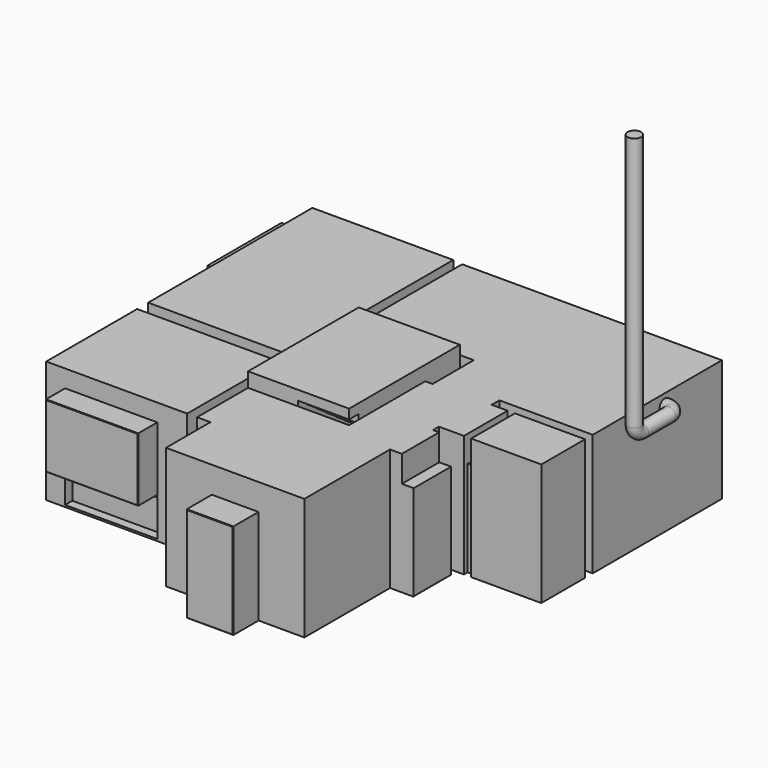
from build123d import *

# Parameters (mm, degrees)
F0_W          = 3096
F0_H          = 4507
F1_DEPTH      = 2680
F2_W          = 2025
F2_H          = 1400
F3_DEPTH      = 532
F4_W          = 2025
F4_H          = 1400
F5_DEPTH      = 532
F6_W          = 2025
F6_H          = 800
F7_DEPTH      = 200
F8_W          = 2700
F8_H          = 303
F9_DEPTH      = 2100
F11_DEPTH     = 2680
F12_W         = 219
F12_H         = 1346
F13_DEPTH     = 2100
F14_W         = 2025
F14_H         = 1400
F15_DEPTH     = 532
F17_DEPTH     = 2680
F18_W         = 1025
F18_H         = 698
F19_DEPTH     = 2100
F21_DEPTH     = 3000
F23_DEPTH     = 1110
F25_DEPTH     = 1120
F27_DEPTH     = 2680
F28_W         = 2000
F28_H         = 1400
F29_DEPTH     = 532
F30_W         = 825
F30_H         = 2100
F31_DEPTH     = 160
F32_W         = 1200
F32_H         = 2680
F33_DEPTH     = 1540
F36_W         = 1025
F36_H         = 2100
F37_DEPTH     = 260
F38_SIZE      = 10
F39_SIZE      = 10
F41_T1_DEPTH  = 2076.4336597593
F41_T3_DEPTH  = 2076.4336597593
F41_T5_DEPTH  = 2051.4336597593
F41_T7_DEPTH  = 1076.4336597593
F41_T9_DEPTH  = 1451.4336597593
F41_T11_DEPTH = 1451.4336597593
F41_T13_DEPTH = 2076.4336597593
F41_T15_DEPTH = 1441.4336597593
F41_T17_DEPTH = 2047.5714172042
F41_T19_DEPTH = 2141.4336597593
F41_T21_DEPTH = 1076.4336597593
F42_W         = 2025
F42_H         = 30
F43_DEPTH     = 200
F44_W         = 2000
F44_H         = 30
F45_DEPTH     = 200
F46_W         = 2025
F46_H         = 30
F47_DEPTH     = 180
F40_W         = 2025
F40_H         = 800
F49_DEPTH     = 200
F50_W         = 2025
F50_H         = 30
F51_DEPTH     = 200
F52_W         = 2025
F52_H         = 800
F53_DEPTH     = 200
F54_W         = 2000
F54_H         = 800
F55_DEPTH     = 200
F48_R         = 150


# Not quite as in the source:
# - a fillet or chamfer that OpenCascade refuses, or shapes differently, is made with other operations: its cross-section is extruded or revolved along the edge and cut away or added


with BuildPart() as f1:
    # F0 (on Top) → F1 (new body)
    with BuildSketch(Plane.XY):
        with Locations((-1.1402405798, 1181.2281365744)):
            Rectangle(F0_W, F0_H)
    extrude(amount=F1_DEPTH)

    # F2 (on face) → F3 (join)
    with BuildSketch(Plane(origin=(0, 3434.7281365744, 0), x_dir=(-1, 0, 0), z_dir=(0, 1, 0))):
        with Locations((-1.3597594202, 1600)):
            Rectangle(F2_W, F2_H)
    extrude(amount=F3_DEPTH)

    # F4 (on face) → F5 (join)
    with BuildSketch(Plane(origin=(-1549.1402405798, 0, 0), x_dir=(0, -1, 0), z_dir=(-1, 0, 0))):
        with Locations((-2226.2281365744, 1600)):
            Rectangle(F4_W, F4_H)
    extrude(amount=F5_DEPTH)

    # F6 (on face) → F7 (cut)
    with BuildSketch(Plane(origin=(0, 3434.7281365744, 0), x_dir=(-1, 0, 0), z_dir=(0, 1, 0))):
        with Locations((-1.3597594202, 435)):
            Rectangle(F6_W, F6_H)
    extrude(amount=-F7_DEPTH, mode=Mode.SUBTRACT)

    # F8 (on face) → F9 (join)
    with BuildSketch(Plane(origin=(0, 0, 0), x_dir=(1, 0, 0), z_dir=(0, 0, -1))):
        with Locations((-1.1402405798, 1223.7718634256)):
            Rectangle(F8_W, F8_H)
    extrude(amount=-F9_DEPTH)

    # F10 (on face) → F11 (join)
    with BuildSketch(Plane(origin=(0, 0, 0), x_dir=(1, 0, 0), z_dir=(0, 0, -1))):
        Polygon((-1549.1402405798, 3872.2718634256), (-1549.1402405798, 1375.2718634256), (-1351.1402405798, 1375.2718634256), (1546.8597594202, 1375.2718634256), (1546.8597594202, 3872.2718634256), align=None)
    extrude(amount=-F11_DEPTH)

    # F12 (on face) → F13 (join)
    with BuildSketch(Plane(origin=(0, 0, 0), x_dir=(1, 0, 0), z_dir=(0, 0, -1))):
        with Locations((1656.3597594202, 3199.2718634256)):
            Rectangle(F12_W, F12_H)
    extrude(amount=-F13_DEPTH)

    # F14 (on face) → F15 (join)
    with BuildSketch(Plane.XZ.offset(3872.2718634256)):
        with Locations((-121.6547704638, 1596.5273075876)):
            Rectangle(F14_W, F14_H)
    extrude(amount=F15_DEPTH)

    # F16 (on face) → F17 (join)
    with BuildSketch(Plane(origin=(0, 0, 0), x_dir=(1, 0, 0), z_dir=(0, 0, -1))):
        Polygon((2057.8597594202, 3872.2718634256), (1765.8597594202, 3872.2718634256), (1765.8597594202, 2526.2718634256), (1765.8597594202, 2474.2718634256), (2915.8597594202, 2474.2718634256), (2915.8597594202, 2739.2718634256), (5096.8597594202, 2739.2718634256), (5096.8597594202, 5091.2718634256), (2057.8597594202, 5091.2718634256), align=None)
    extrude(amount=-F17_DEPTH)

    # F18 (on face) → F19 (join)
    with BuildSketch(Plane(origin=(0, 0, 0), x_dir=(1, 0, 0), z_dir=(0, 0, -1))):
        with Locations((3577.3597594202, 5440.2718634256)):
            Rectangle(F18_W, F18_H)
    extrude(amount=-F19_DEPTH)

    # F20 (on face) → F21 (join)
    with BuildSketch(Plane(origin=(0, 0, 0), x_dir=(1, 0, 0), z_dir=(0, 0, -1))):
        Polygon((2915.8597594202, 2474.2718634256), (1765.8597594202, 2474.2718634256), (1765.8597594202, -565.7281365744), (3985.8597594202, -565.7281365744), (3985.8597594202, 2474.2718634256), align=None)
    extrude(amount=-F21_DEPTH)

    # F22 (on face) → F23 (cut)
    with BuildSketch(Plane(origin=(1765.8597594202, 0, 0), x_dir=(0, -1, 0), z_dir=(-1, 0, 0))):
        Polygon((1199.2718634256, 850), (1199.2718634256, 1020), (944.2718634256, 1020), (944.2718634256, 1190), (689.2718634256, 1190), (689.2718634256, 1330), (434.2718634256, 1330), (434.2718634256, 1530), (-565.7281365744, 1530), (-565.7281365744, 1330), (179.2718634256, 1330), (2219.2718634256, 0), (2474.2718634256, 0), (2474.2718634256, 170), (2219.2718634256, 170), (2219.2718634256, 340), (1964.2718634256, 340), (1964.2718634256, 510), (1709.2718634256, 510), (1709.2718634256, 680), (1454.2718634256, 680), (1454.2718634256, 850), align=None)
    extrude(amount=-F23_DEPTH, mode=Mode.SUBTRACT)

    # F24 (on face) → F25 (cut)
    with BuildSketch(Plane.YZ.offset(3985.8597594202)):
        Polygon((565.7281365744, 1330), (565.7281365744, 1530), (-689.2718634256, 1530), (-689.2718634256, 1710), (-944.2718634256, 1710), (-944.2718634256, 1890), (-1199.2718634256, 1890), (-1199.2718634256, 2070), (-1454.2718634256, 2070), (-1454.2718634256, 2250), (-1709.2718634256, 2250), (-1709.2718634256, 2430), (-1964.2718634256, 2430), (-1964.2718634256, 2610), (-2219.2718634256, 2610), (-2219.2718634256, 2790), (-2474.2718634256, 2790), (-2474.2718634256, 2651.8891687657), (-689.2718634256, 1330), align=None)
    extrude(amount=-F25_DEPTH, mode=Mode.SUBTRACT)

    # F26 (on face) → F27 (join)
    with BuildSketch(Plane.XY.offset(2680)):
        Polygon((2915.8597594202, -2739.2718634256), (5096.8597594202, -2739.2718634256), (5356.8597594202, -2739.2718634256), (5356.8597594202, -1714.2718634256), (5221.8597594202, -1714.2718634256), (5221.8597594202, -1554.2718634256), (5771.8597594202, -1554.2718634256), (5771.8597594202, -1454.2718634256), (5771.8597594202, -629.2718634256), (5771.8597594202, -354.2718634256), (5421.8597594202, -354.2718634256), (5421.8597594202, -142.2718634256), (7471.8597594202, -142.2718634256), (7471.8597594202, 3404.7281365744), (6893.8597594202, 3404.7281365744), (4681.8597594202, 3404.7281365744), (1765.8597594202, 3404.7281365744), (1765.8597594202, 747.7281365744), (4146.8597594202, 747.7281365744), (4146.8597594202, -384.2718634256), (3985.8597594202, -384.2718634256), (3985.8597594202, -2474.2718634256), (2915.8597594202, -2474.2718634256), align=None)
    extrude(amount=-F27_DEPTH)

    # F28 (on face) → F29 (join)
    with BuildSketch(Plane(origin=(0, 3404.7281365744, 0), x_dir=(-1, 0, 0), z_dir=(0, 1, 0))):
        with Locations((-5883.8597594202, 1600)):
            Rectangle(F28_W, F28_H)
    extrude(amount=F29_DEPTH)

    # F30 (on face) → F31 (join)
    with BuildSketch(Plane.YZ.offset(5771.8597594202)):
        with Locations((-1041.7718634256, 1050)):
            Rectangle(F30_W, F30_H)
    extrude(amount=F31_DEPTH)

    # F32 (on face) → F33 (join)
    with BuildSketch(Plane.YZ.offset(5931.8597594202)):
        with Locations((-954.2718634256, 1340)):
            Rectangle(F32_W, F32_H)
    extrude(amount=F33_DEPTH)

    # F34: union 

    # F36 (on face) → F37 (join)
    with BuildSketch(Plane.YZ.offset(5356.8597594202)):
        with Locations((-2226.7718634256, 1050)):
            Rectangle(F36_W, F36_H)
    extrude(amount=F37_DEPTH)

    # F38
    f38_edges = [f1.edges().sort_by_distance(p)[0] for p in [
        (1.359759, 3966.728137, 900),
    ]]
    chamfer(f38_edges, length=F38_SIZE)

    # F39
    f39_edges = [f1.edges().sort_by_distance(p)[0] for p in [
        (3577.359759, -5789.271863, 0),
    ]]
    chamfer(f39_edges, length=F39_SIZE)

    # F41: chamfer of 10 on 20 edges, made by hand

    # F41_s2 → F41_t1 (cut)
    with BuildSketch(Plane.YZ.offset(-1159.8716003435)):
        Polygon((-4394.2718634256, 896.5273075876), (-4404.2718634256, 906.5273075876), (-4404.2718634256, 896.5273075876), align=None)
        Polygon((-4394.2718634256, 2296.5273075876), (-4404.2718634256, 2286.5273075876), (-4404.2718634256, 2296.5273075876), align=None)
    extrude(amount=F41_T1_DEPTH, mode=Mode.SUBTRACT)

    # F41_s4 → F41_t3 (cut)
    with BuildSketch(Plane.XZ.offset(-3264.4449664541)):
        Polygon((-2071.1402405798, 900), (-2081.1402405798, 910), (-2081.1402405798, 900), align=None)
        Polygon((-2071.1402405798, 2300), (-2081.1402405798, 2290), (-2081.1402405798, 2300), align=None)
    extrude(amount=F41_T3_DEPTH, mode=Mode.SUBTRACT)

    # F41_s6 → F41_t5 (cut)
    with BuildSketch(Plane.YZ.offset(4858.1429295405)):
        Polygon((3926.7281365744, 900), (3936.7281365744, 910), (3936.7281365744, 900), align=None)
        Polygon((3926.7281365744, 2300), (3936.7281365744, 2290), (3936.7281365744, 2300), align=None)
    extrude(amount=F41_T5_DEPTH, mode=Mode.SUBTRACT)

    # F41_s8 → F41_t7 (cut)
    with BuildSketch(Plane.XZ.offset(1688.5550335459)):
        Polygon((5606.8597594202, 0), (5616.8597594202, 10), (5616.8597594202, 0), align=None)
    extrude(amount=F41_T7_DEPTH, mode=Mode.SUBTRACT)

    # F41_s10 → F41_t9 (cut)
    with BuildSketch(Plane.XY.offset(870.8104777079)):
        Polygon((-1134.1547704638, -4394.2718634256), (-1124.1547704638, -4404.2718634256), (-1134.1547704638, -4404.2718634256), align=None)
        Polygon((890.8452295362, -4394.2718634256), (880.8452295362, -4404.2718634256), (890.8452295362, -4404.2718634256), align=None)
    extrude(amount=F41_T9_DEPTH, mode=Mode.SUBTRACT)

    # F41_s12 → F41_t11 (cut)
    with BuildSketch(Plane.XY.offset(874.2831701203)):
        Polygon((-2071.1402405798, 1213.7281365744), (-2081.1402405798, 1223.7281365744), (-2081.1402405798, 1213.7281365744), align=None)
        Polygon((-2071.1402405798, 3238.7281365744), (-2081.1402405798, 3228.7281365744), (-2081.1402405798, 3238.7281365744), align=None)
        Polygon((4883.8597594202, 3926.7281365744), (4893.8597594202, 3936.7281365744), (4883.8597594202, 3936.7281365744), align=None)
        Polygon((6883.8597594202, 3926.7281365744), (6873.8597594202, 3936.7281365744), (6883.8597594202, 3936.7281365744), align=None)
    extrude(amount=F41_T11_DEPTH, mode=Mode.SUBTRACT)

    # F41_s14 → F41_t13 (cut)
    with BuildSketch(Plane.YZ.offset(-1036.8570704595)):
        Polygon((3956.7281365744, 2300), (3966.7281365744, 2290), (3966.7281365744, 2300), align=None)
    extrude(amount=F41_T13_DEPTH, mode=Mode.SUBTRACT)

    # F41_s16 → F41_t15 (cut)
    with BuildSketch(Plane.XY.offset(884.2831701203)):
        Polygon((1013.8597594202, 3956.7281365744), (1003.8597594202, 3966.7281365744), (1013.8597594202, 3966.7281365744), align=None)
        Polygon((-1011.1402405798, 3956.7281365744), (-1001.1402405798, 3966.7281365744), (-1011.1402405798, 3966.7281365744), align=None)
    extrude(amount=F41_T15_DEPTH, mode=Mode.SUBTRACT)

    # F41_s18 → F41_t17 (cut)
    with BuildSketch(Plane.YZ.offset(-1022.425949182)):
        Polygon((3963.7992043863, 907.0710678119), (3966.7281365744, 914.1421356237), (3966.7281365744, 910), align=None)
    extrude(amount=F41_T17_DEPTH, mode=Mode.SUBTRACT)

    # F41_s20 → F41_t19 (cut)
    with BuildSketch(Plane.XY.offset(-15.7168298797)):
        Polygon((3064.8597594202, -5779.2718634256), (3074.8597594202, -5789.2718634256), (3064.8597594202, -5789.2718634256), align=None)
        Polygon((4089.8597594202, -5779.2718634256), (4079.8597594202, -5789.2718634256), (4089.8597594202, -5789.2718634256), align=None)
    extrude(amount=F41_T19_DEPTH, mode=Mode.SUBTRACT)

    # F41_s22 → F41_t21 (cut)
    with BuildSketch(Plane.YZ.offset(3039.1429295405)):
        Polygon((-5789.2718634256, 2090), (-5779.2718634256, 2100), (-5789.2718634256, 2100), align=None)
    extrude(amount=F41_T21_DEPTH, mode=Mode.SUBTRACT)

    # F42 (on face) → F43 (cut)
    with BuildSketch(Plane(origin=(0, 3434.7281365744, 0), x_dir=(-1, 0, 0), z_dir=(0, 1, 0))):
        with Locations((-1.3597594202, 885)):
            Rectangle(F42_W, F42_H)
    extrude(amount=-F43_DEPTH, mode=Mode.SUBTRACT)

    # F44 (on face) → F45 (cut)
    with BuildSketch(Plane(origin=(0, 3404.7281365744, 0), x_dir=(-1, 0, 0), z_dir=(0, 1, 0))):
        with Locations((-5883.8597594202, 885)):
            Rectangle(F44_W, F44_H)
    extrude(amount=-F45_DEPTH, mode=Mode.SUBTRACT)

    # F46 (on face) → F47 (cut)
    with BuildSketch(Plane.XZ.offset(3872.2718634256)):
        with Locations((-121.6547704638, 881.5273075876)):
            Rectangle(F46_W, F46_H)
    extrude(amount=-F47_DEPTH, mode=Mode.SUBTRACT)

    # F40 (on face) → F49 (cut)
    with BuildSketch(Plane(origin=(-1549.1402405798, 0, 0), x_dir=(0, -1, 0), z_dir=(-1, 0, 0))):
        with Locations((-2226.2281365744, 460)):
            Rectangle(F40_W, F40_H)
    extrude(amount=-F49_DEPTH, mode=Mode.SUBTRACT)

    # F50 (on face) → F51 (cut)
    with BuildSketch(Plane(origin=(-1549.1402405798, 0, 0), x_dir=(0, -1, 0), z_dir=(-1, 0, 0))):
        with Locations((-2226.2281365744, 885)):
            Rectangle(F50_W, F50_H)
    extrude(amount=-F51_DEPTH, mode=Mode.SUBTRACT)

    # F52 (on face) → F53 (cut)
    with BuildSketch(Plane.XZ.offset(3872.2718634256)):
        with Locations((-121.6547704638, 441.5273075876)):
            Rectangle(F52_W, F52_H)
    extrude(amount=-F53_DEPTH, mode=Mode.SUBTRACT)

    # F54 (on face) → F55 (cut)
    with BuildSketch(Plane(origin=(0, 3404.7281365744, 0), x_dir=(-1, 0, 0), z_dir=(0, 1, 0))):
        with Locations((-5883.8597594202, 445)):
            Rectangle(F54_W, F54_H)
    extrude(amount=-F55_DEPTH, mode=Mode.SUBTRACT)

    # F60: sweep along a path in F57, F59
    with BuildLine(Plane.XY.offset(2430)) as f60_path:
        Line((7471.8597594202, 1837.7281365744), (7521.8597594202, 1837.7281365744))
        ThreePointArc((7521.8597594202, 1837.7281365744), (7663.2811156575, 1779.1494928117), (7721.8597594202, 1637.7281365744))
    with BuildLine(Plane.YZ.offset(7721.8597594202)) as f60_path_2:
        Line((1637.7281365744, 2430), (887.7281365744, 2430))
        ThreePointArc((887.7281365744, 2430), (746.3067803371, 2488.5786437627), (687.7281365744, 2630))
        Line((687.7281365744, 2630), (687.7281365744, 8230))
    # F48 (on face) → F60 (sweep)
    with BuildSketch(Plane.YZ.offset(7471.8597594202)):
        with Locations((1837.7281365744, 2430)):
            Circle(F48_R)
    sweep(path=f60_path.line + f60_path_2.line)


solid = f1.part
